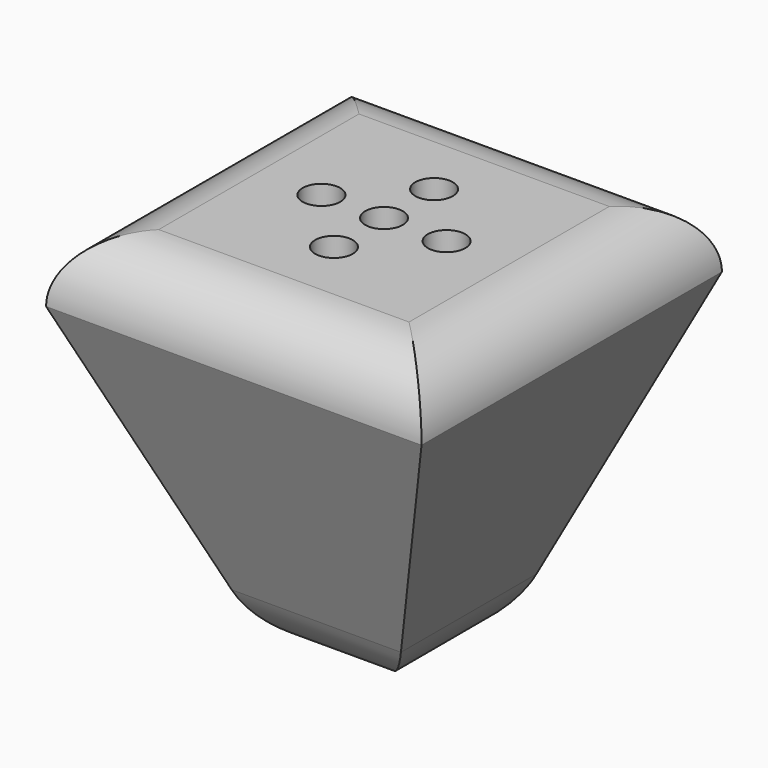
from build123d import *

# Parameters (mm, degrees)
F0_W     = 60
F0_H     = 60
F1_DEPTH = 60
F3_D     = 6
F3_DEPTH = 10
F3_TIP   = 1.8025818571
F4_SIZE2 = 50
F4_SIZE  = 20
F5_R     = 14
F6_R     = 9.99999


# Not quite as in the source:
# - a fillet or chamfer is up to 0.001 mm smaller than in the source, because OpenCascade refuses the exact size


with BuildPart() as f1:
    # F0 (on Top) → F1 (new body)
    with BuildSketch(Plane.XY):
        Rectangle(F0_W, F0_H)
    extrude(amount=F1_DEPTH)

    # F3
    with Locations(Plane.XY.offset(60)):
        with Locations((0, 10), (-10, 0), (10, 0), (0, -10), (0, 0)):
            Hole(F3_D / 2, depth=F3_DEPTH)
            with Locations((0, 0, -(F3_DEPTH + F3_TIP / 2))):  # 118° drill point
                Cone(0, F3_D / 2, F3_TIP, mode=Mode.SUBTRACT)

    # F4
    f4_edges = [f1.edges().sort_by_distance(p)[0] for p in [
        (-30, 0, 0),
        (0, -30, 0),
        (30, 0, 0),
        (0, 30, 0),
    ]]
    f4_side = f1.faces().sort_by_distance((0, 0, 0))[0]
    chamfer(f4_edges, length=F4_SIZE, length2=F4_SIZE2, reference=f4_side)

    # F5
    f5_edges = [f1.edges().sort_by_distance(p)[0] for p in [
        (-10, 0, 0),
        (0, 10, 0),
        (0, -10, 0),
        (10, 0, 0),
    ]]
    fillet(f5_edges, radius=F5_R)

    # F6 (radius 10 in the source; OpenCascade refuses exactly that, so slightly less here)
    f6_edges = [f1.edges().sort_by_distance(p)[0] for p in [
        (-30, 0, 60),
        (0, 30, 60),
        (30, 0, 60),
        (0, -30, 60),
    ]]
    fillet(f6_edges, radius=F6_R)


solid = f1.part
